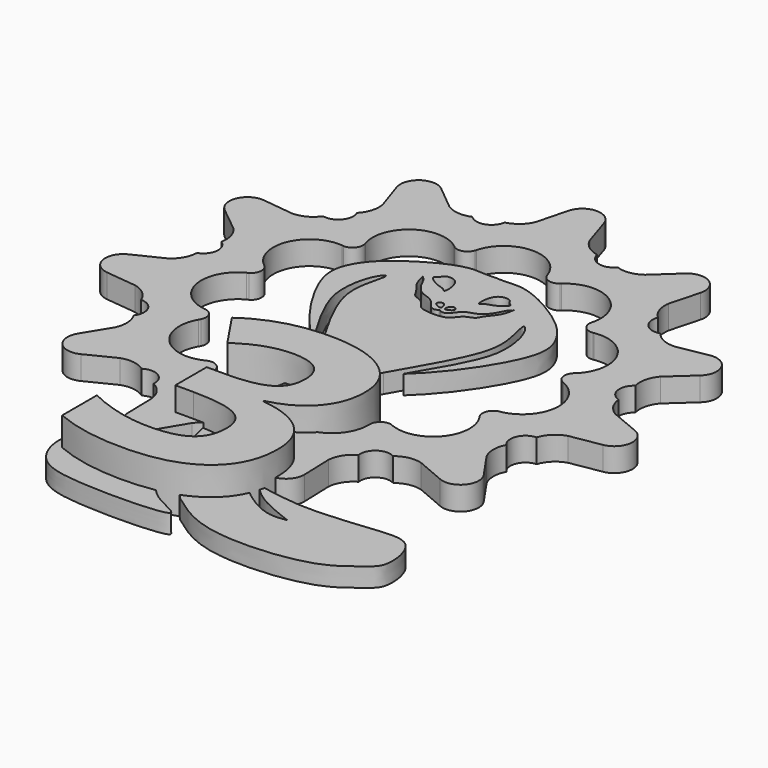
from build123d import *

# Parameters (mm, degrees)
F1_DEPTH     = 5
F3_DEPTH     = 4
F4_TEXT_SIZE = 71.6005038056
F5_DEPTH     = 10


# Not quite as in the source:
# - Text() gives the source's letters only with a copy of the font that has no kerning and outlines rounded to 1/6400 em; it was checked with that copy


with BuildPart() as f1:
    # F0 (on Top) → F1 (new body)
    with BuildSketch(Plane.XY):
        with BuildLine():
            ThreePointArc((-117.2096186083, -24.8238547917), (-113.9793205084, -29.5817996447), (-109.6649228447, -25.7793217897))
            ThreePointArc((-109.6649228447, -25.7793217897), (-109.7109933352, -25.1868355634), (-109.8480972803, -24.6085925984))
            ThreePointArc((-109.8480972803, -24.6085925984), (-113.6098018142, -21.9481109336), (-117.2096186083, -24.8238547917))
        make_face()
        with BuildLine():
            ThreePointArc((-109.8480972803, -24.6085925984), (-109.7109933352, -25.1868355634), (-109.6649228447, -25.7793217897))
            ThreePointArc((-109.6649228447, -25.7793217897), (-113.9793205084, -29.5817996447), (-117.2096186083, -24.8238547917))
            Line((-117.2096186083, -24.8238547917), (-118.8519075513, -31.2039032578))
            ThreePointArc((-118.8519075513, -31.2039032578), (-120.3942965539, -33.4215473324), (-122.7970570326, -34.6559099853))
            ThreePointArc((-122.7970570326, -34.6559099853), (-124.9522527799, -37.2281972482), (-128.2088887321, -36.4183498881))
            ThreePointArc((-128.2088887321, -36.4183498881), (-130.877743488, -36.8356308111), (-133.4302536555, -35.9515488457))
            Line((-133.4302536555, -35.9515488457), (-138.51463756, -31.7621369879))
            ThreePointArc((-138.51463756, -31.7621369879), (-143.1175497707, -31.5577284026), (-144.591163856, -35.923165977))
            Line((-144.591163856, -35.923165977), (-142.5234306131, -42.1782927254))
            ThreePointArc((-142.5234306131, -42.1782927254), (-142.6220219053, -44.8777720889), (-143.9760058128, -47.2152144208))
            ThreePointArc((-143.9760058128, -47.2152144208), (-144.3983883606, -50.5443469588), (-147.5758813994, -51.6237303294))
            ThreePointArc((-147.5758813994, -51.6237303294), (-149.595465792, -53.417661197), (-152.2207447845, -54.0539153038))
            Line((-152.2207447845, -54.0539153038), (-158.7629677579, -53.2783832483))
            ThreePointArc((-158.7629677579, -53.2783832483), (-162.7456955411, -55.594946024), (-161.6252448576, -60.0640817296))
            Line((-161.6252448576, -60.0640817296), (-156.5039801235, -64.2083282143))
            ThreePointArc((-156.5039801235, -64.2083282143), (-155.1274716666, -66.5325772424), (-155.0027986791, -69.2309778285))
            ThreePointArc((-155.0027986791, -69.2309778285), (-153.558264553, -72.2599795833), (-155.6477830895, -74.885897091))
            ThreePointArc((-155.6477830895, -74.885897091), (-156.376893344, -77.486917528), (-158.2414336307, -79.4415015236))
            Line((-158.2414336307, -79.4415015236), (-164.164386104, -82.3260752185))
            ThreePointArc((-164.164386104, -82.3260752185), (-166.2624415292, -86.428117042), (-162.9036612522, -89.5820318695))
            Line((-162.9036612522, -89.5820318695), (-156.3548303948, -90.2996291135))
            ThreePointArc((-156.3548303948, -90.2996291135), (-153.9402538979, -91.5107151622), (-152.3765068081, -93.7133508823))
            ThreePointArc((-152.3765068081, -93.7133508823), (-149.5236853864, -95.4805351987), (-149.8618220492, -98.8192765887))
            ThreePointArc((-149.8618220492, -98.8192765887), (-149.0689708113, -101.4015809842), (-149.5807940254, -104.0539282605))
            Line((-149.5807940254, -104.0539282605), (-153.003980438, -109.682775939))
            ThreePointArc((-153.003980438, -109.682775939), (-152.5512457318, -114.267927515), (-148.0205248672, -115.1052757913))
            Line((-148.0205248672, -115.1052757913), (-142.123335412, -112.1683917398))
            ThreePointArc((-142.123335412, -112.1683917398), (-139.4373018523, -111.8818035458), (-136.9309593122, -112.8893531219))
            ThreePointArc((-136.9309593122, -112.8893531219), (-133.5756012393, -112.8336514657), (-132.0550000271, -115.8251899371))
            ThreePointArc((-132.0550000271, -115.8251899371), (-129.9919119629, -117.5689148913), (-128.9885178503, -120.0769239287))
            Line((-128.9885178503, -120.0769239287), (-128.8251007032, -126.6629262244))
            ThreePointArc((-128.8251007032, -126.6629262244), (-125.965315936, -130.2754343246), (-121.7011263458, -128.5303638883))
            Line((-121.7011263458, -128.5303638883), (-118.3278942772, -122.8714384767))
            ThreePointArc((-118.3278942772, -122.8714384767), (-116.2232003313, -121.1781657666), (-113.5700083885, -120.6707393274))
            ThreePointArc((-113.5700083885, -120.6707393274), (-110.7774161447, -118.8098365809), (-107.8808571983, -120.5043798061))
            ThreePointArc((-107.8808571983, -120.5043798061), (-105.2025481911, -120.8559049667), (-103.0025072929, -122.4233006165))
            Line((-103.0025072929, -122.4233006165), (-99.3043703757, -127.8754483349))
            ThreePointArc((-99.3043703757, -127.8754483349), (-94.9454970048, -129.3683671623), (-92.3016887545, -125.594925547))
            Line((-92.3016887545, -125.594925547), (-92.5233914202, -119.0106276094))
            ThreePointArc((-92.5233914202, -119.0106276094), (-91.6682625448, -116.4482725046), (-89.7105908946, -114.586974359))
            ThreePointArc((-89.7105908946, -114.586974359), (-88.3673927857, -111.5116939958), (-85.0145131046, -111.371236474))
            ThreePointArc((-85.0145131046, -111.371236474), (-82.5713273401, -110.2189550861), (-79.8731370967, -110.3481003042))
            Line((-79.8731370967, -110.3481003042), (-73.8144127508, -112.9353750679))
            ThreePointArc((-73.8144127508, -112.9353750679), (-69.3403622731, -111.8347134433), (-69.156325802, -107.2309416998))
            Line((-69.156325802, -107.2309416998), (-72.9025741721, -101.811739309))
            ThreePointArc((-72.9025741721, -101.811739309), (-73.5685077432, -99.1938314505), (-72.9279033022, -96.5696106086))
            ThreePointArc((-72.9279033022, -96.5696106086), (-73.4605552373, -93.2563324151), (-70.7158704298, -91.325468417))
            ThreePointArc((-70.7158704298, -91.325468417), (-69.2835021255, -89.0352216797), (-66.9438188747, -87.6851137718))
            Line((-66.9438188747, -87.6851137718), (-60.4481092711, -86.5860741241))
            ThreePointArc((-60.4481092711, -86.5860741241), (-57.2793611012, -83.2412843363), (-59.6135266884, -79.2688474646))
            Line((-59.6135266884, -79.2688474646), (-65.6949133751, -76.7352990894))
            ThreePointArc((-65.6949133751, -76.7352990894), (-67.6704801891, -74.893005725), (-68.5503303411, -72.3390337622))
            ThreePointArc((-68.5503303411, -72.3390337622), (-70.7897190943, -69.8397001543), (-69.5246471938, -66.7314653564))
            ThreePointArc((-69.5246471938, -66.7314653564), (-69.5578631658, -64.0303904267), (-68.3195198083, -61.6296791142))
            Line((-68.3195198083, -61.6296791142), (-63.4491668495, -57.1932623778))
            ThreePointArc((-63.4491668495, -57.1932623778), (-62.591776142, -52.6662915513), (-66.7030627062, -50.5864101902))
            Line((-66.7030627062, -50.5864101902), (-73.1887904055, -51.7428995386))
            ThreePointArc((-73.1887904055, -51.7428995386), (-75.8467619576, -51.2611357945), (-77.967720496, -49.5882807635))
            ThreePointArc((-77.967720496, -49.5882807635), (-81.202855961, -48.6964125022), (-81.8190483573, -45.3976494912))
            ThreePointArc((-81.8190483573, -45.3976494912), (-83.3073027691, -43.1433185744), (-83.5634645712, -40.4542127364))
            Line((-83.5634645712, -40.4542127364), (-81.8647709095, -34.0889498788))
            ThreePointArc((-81.8647709095, -34.0889498788), (-83.590953156, -29.8170792651), (-88.1740562618, -30.290101051))
            Line((-88.1740562618, -30.290101051), (-93.0049522552, -34.7694509261))
            ThreePointArc((-93.0049522552, -34.7694509261), (-95.501441358, -35.8011733872), (-98.1901189329, -35.5405549404))
            ThreePointArc((-98.1901189329, -35.5405549404), (-101.3938684578, -36.5393138971), (-103.695688419, -34.097356621))
            ThreePointArc((-103.695688419, -34.097356621), (-106.1664710103, -33.0055038548), (-107.8358084098, -30.8817755946))
            Line((-107.8358084098, -30.8817755946), (-109.8480972803, -24.6085925984))
        make_face()
        with BuildLine():
            ThreePointArc((-120.2761988919, -45.2671052015), (-113.1332584373, -39.6167331027), (-105.6182130227, -44.7618662992))
            ThreePointArc((-105.6182130227, -44.7618662992), (-105.5515166298, -44.9618399206), (-105.4903344746, -45.1635689516))
            ThreePointArc((-105.4903344746, -45.1635689516), (-103.9595719314, -46.4625857559), (-102.0028203403, -46.0133621674))
            ThreePointArc((-102.0028203403, -46.0133621674), (-101.9053533079, -45.9208909988), (-101.8062833721, -45.8301392094))
            ThreePointArc((-101.8062833721, -45.8301392094), (-93.5450584899, -44.5228398864), (-88.990003067, -51.5377053996))
            ThreePointArc((-88.990003067, -51.5377053996), (-89.0431986034, -52.4400086199), (-89.2020482023, -53.3298106605))
            ThreePointArc((-89.2020482023, -53.3298106605), (-89.2540535283, -53.5340979684), (-89.3116467723, -53.7368807988))
            ThreePointArc((-89.3116467723, -53.7368807988), (-88.7261888819, -55.6572759873), (-86.8371960849, -56.3372648362))
            ThreePointArc((-86.8371960849, -56.3372648362), (-86.7052079114, -56.312167795), (-86.5728008563, -56.2893837827))
            ThreePointArc((-86.5728008563, -56.2893837827), (-80.3630657899, -58.0177108599), (-77.6577832051, -63.8682980284))
            ThreePointArc((-77.6577832051, -63.8682980284), (-78.2740870509, -66.882499127), (-80.024071995, -69.4128728916))
            ThreePointArc((-80.024071995, -69.4128728916), (-80.1782677164, -69.5566141091), (-80.3363509116, -69.6960686231))
            ThreePointArc((-80.3363509116, -69.6960686231), (-80.8820764175, -71.6281302923), (-79.6605842807, -73.2214399236))
            ThreePointArc((-79.6605842807, -73.2214399236), (-79.5359802785, -73.2716851431), (-79.4122744087, -73.3241026707))
            ThreePointArc((-79.4122744087, -73.3241026707), (-76.0493885489, -76.1557842028), (-74.79093489, -80.368113249))
            ThreePointArc((-74.79093489, -80.368113249), (-76.5425275911, -85.250019579), (-80.9982269983, -87.9047943715))
            ThreePointArc((-80.9982269983, -87.9047943715), (-81.2056570629, -87.9423526777), (-81.4140399118, -87.9742030524))
            ThreePointArc((-81.4140399118, -87.9742030524), (-82.9176848218, -89.3045152737), (-82.7515084679, -91.3052811373))
            ThreePointArc((-82.7515084679, -91.3052811373), (-82.6738495275, -91.4149161153), (-82.5981205824, -91.5258929881))
            ThreePointArc((-82.5981205824, -91.5258929881), (-81.6314443255, -93.5657632348), (-81.2996622055, -95.798576311))
            ThreePointArc((-81.2996622055, -95.798576311), (-84.6667499566, -102.1526848554), (-91.8152258815, -102.9345206881))
            ThreePointArc((-91.8152258815, -102.9345206881), (-92.0100327095, -102.8539715861), (-92.2025551299, -102.7681055526))
            ThreePointArc((-92.2025551299, -102.7681055526), (-94.1867228094, -103.0743035952), (-95.1286220566, -104.8472966661))
            ThreePointArc((-95.1286220566, -104.8472966661), (-95.1225643428, -104.9815130717), (-95.1188557274, -105.1158149169))
            ThreePointArc((-95.1188557274, -105.1158149169), (-95.1178316026, -105.1882163487), (-95.1174902175, -105.2606242187))
            ThreePointArc((-95.1174902175, -105.2606242187), (-100.449401412, -112.5721628925), (-109.0407479285, -109.7302199307))
            ThreePointArc((-109.0407479285, -109.7302199307), (-109.1610817285, -109.5571371914), (-109.2766192122, -109.3808166086))
            ThreePointArc((-109.2766192122, -109.3808166086), (-111.1113504424, -108.5656847574), (-112.8622789349, -109.5479922631))
            ThreePointArc((-112.8622789349, -109.5479922631), (-112.929745729, -109.6641773358), (-112.9992349025, -109.7791642664))
            ThreePointArc((-112.9992349025, -109.7791642664), (-121.4447298582, -113.1882577158), (-127.2058115992, -106.1343056061))
            ThreePointArc((-127.2058115992, -106.1343056061), (-127.2134672398, -105.9236417761), (-127.2153374522, -105.7128471832))
            ThreePointArc((-127.2153374522, -105.7128471832), (-128.318118031, -104.0351840417), (-130.3221683439, -103.9149302896))
            ThreePointArc((-130.3221683439, -103.9149302896), (-130.4417394155, -103.9761960899), (-130.5623640564, -104.0353605678))
            ThreePointArc((-130.5623640564, -104.0353605678), (-139.5102615936, -102.3372931793), (-140.5431375262, -93.2884551046))
            ThreePointArc((-140.5431375262, -93.2884551046), (-140.4356843958, -93.1070944616), (-140.3232935575, -92.9287516525))
            ThreePointArc((-140.3232935575, -92.9287516525), (-140.3439984431, -90.9212034142), (-141.964898762, -89.736568121))
            ThreePointArc((-141.964898762, -89.736568121), (-142.0986111407, -89.7234631901), (-142.2320737777, -89.7080209117))
            ThreePointArc((-142.2320737777, -89.7080209117), (-148.8414796513, -83.441917083), (-144.8182189649, -75.2711351962))
            ThreePointArc((-144.8182189649, -75.2711351962), (-144.629772673, -75.1766584628), (-144.4388040811, -75.0873900193))
            ThreePointArc((-144.4388040811, -75.0873900193), (-143.3708596186, -73.3873390652), (-144.093985545, -71.5144355663))
            ThreePointArc((-144.093985545, -71.5144355663), (-144.1993864954, -71.4311206271), (-144.3033136842, -71.3459744067))
            ThreePointArc((-144.3033136842, -71.3459744067), (-146.4757882291, -62.5012778294), (-138.6737477646, -57.8027176474))
            ThreePointArc((-138.6737477646, -57.8027176474), (-138.4641386775, -57.825120519), (-138.2552235106, -57.8532685411))
            ThreePointArc((-138.2552235106, -57.8532685411), (-136.4376945211, -57.0004690372), (-136.0334586827, -55.0339309601))
            ThreePointArc((-136.0334586827, -55.0339309601), (-136.0770841477, -54.9068579172), (-136.1184797403, -54.7790410781))
            ThreePointArc((-136.1184797403, -54.7790410781), (-133.1642776385, -46.1638804218), (-124.0605501168, -46.429301604))
            ThreePointArc((-124.0605501168, -46.429301604), (-123.8963276385, -46.5614713272), (-123.7357949861, -46.6980990168))
            ThreePointArc((-123.7357949861, -46.6980990168), (-121.7457340817, -46.9633087799), (-120.342478501, -45.5274980693))
            ThreePointArc((-120.342478501, -45.5274980693), (-120.3104777038, -45.3970117159), (-120.2761988919, -45.2671052015))
        make_face(mode=Mode.SUBTRACT)
    extrude(amount=F1_DEPTH)

    # F2 (on Top) → F3 (join)
    with BuildSketch(Plane.XY):
        with BuildLine():
            add(Edge.make_bspline(
                [(-112.8318831325, -49.5106913149), (-110.8358390301, -49.7867201321), (-106.8673193815, -48.3627424801), (-95.4730686789, -54.9641453728), (-91.24145791, -59.9110418173), (-88.8182301333, -66.581057202), (-97.3949212358, -80.1979328277), (-101.4951824369, -84.1600654045), (-103.252193262, -85.8743322902)],
                knots=[0, 0, 0, 0, 0.1365349459, 0.3342831137, 0.4785284841, 0.6175654811, 0.8376307999, 1, 1, 1, 1], degree=3))
            add(Edge.make_bspline(
                [(-112.8318831325, -49.5106913149), (-114.8279272348, -49.7867201321), (-118.7964468834, -48.3627424801), (-130.190697586, -54.9641453728), (-134.4223083549, -59.9110418173), (-136.8455361317, -66.581057202), (-128.2688450291, -80.1979328277), (-124.168583828, -84.1600654045), (-122.4115730029, -85.8743322902)],
                knots=[0, 0, 0, 0, 0.1365349459, 0.3342831137, 0.4785284841, 0.6175654811, 0.8376307999, 1, 1, 1, 1], degree=3))
            add(Edge.make_bspline(
                [(-122.4115730029, -85.8743322902), (-124.958112917, -81.6141024189), (-129.2089516234, -74.369457322), (-130.4225910024, -68.1737151841), (-129.3185920534, -62.1735759595), (-126.9601199795, -59.2936404783), (-127.8236442382, -63.3904845171), (-129.9288002995, -70.947818882), (-118.5329024032, -88.3060464577), (-114.9407244822, -98.0306761721), (-119.7444756613, -110.6590313317), (-116.479102874, -126.0767500088), (-113.2716186955, -132.3290730332), (-112.8318831325, -133.1038787181)],
                knots=[0, 0, 0, 0, 0.1073418359, 0.1800553274, 0.2527196236, 0.2951183014, 0.3404049451, 0.4217451234, 0.5528269749, 0.6458771787, 0.7495835625, 0.8817656203, 0.9014576568, 0.9014576568, 0.9014576568, 0.9014576568], degree=3))
            add(Edge.make_bspline(
                [(-106.4971447376, -88.3240836838), (-106.5080314354, -88.3443907053), (-108.561729288, -92.1796397896), (-110.7230417827, -98.0306761721), (-105.9192906036, -110.6590313317), (-109.184663391, -126.0767500088), (-112.3921475694, -132.3290730332), (-112.8318831325, -133.1038787181)],
                knots=[0.5523323878, 0.5523323878, 0.5523323878, 0.5523323878, 0.5528269749, 0.6458771787, 0.7495835625, 0.8817656203, 0.9014576568, 0.9014576568, 0.9014576568, 0.9014576568], degree=3))
            add(Edge.make_bspline(
                [(-106.1023806814, -87.5969630464), (-106.247526419, -87.8281931787), (-106.3789975954, -88.0715097531), (-106.4971447376, -88.3240836838)],
                knots=[0, 0, 0, 0, 0.0668727136, 0.0668727136, 0.0668727136, 0.0668727136], degree=3))
            add(Edge.make_bspline(
                [(-103.252193262, -85.8743322902), (-100.7056533479, -81.6141024189), (-96.4548146415, -74.369457322), (-95.2411752625, -68.1737151841), (-96.3451742116, -62.1735759595), (-98.7036462854, -59.2936404783), (-97.8401220267, -63.3904845171), (-95.7864452579, -70.763012523), (-103.1978484029, -82.3074697159), (-106.1023806814, -87.5969630464)],
                knots=[0, 0, 0, 0, 0.1073418359, 0.1800553274, 0.2527196236, 0.2951183014, 0.3404049451, 0.4217451234, 0.5465249907, 0.5465249907, 0.5465249907, 0.5465249907], degree=3))
        make_face()
        with BuildLine():
            add(Edge.make_bspline(
                [(-120.9213361144, -55.7986162603), (-120.9253523737, -55.5501994682), (-120.121301053, -55.2735206681), (-119.914520435, -54.0254688498), (-116.3753834879, -53.9011755123), (-116.1277862601, -59.2035980251), (-117.1620053446, -57.8149655297), (-118.6804147561, -57.7393391349), (-120.9141481965, -56.2432089485), (-120.9213361144, -55.7986162603)],
                knots=[0, 0, 0, 0, 0.0989707847, 0.2106465985, 0.3821345415, 0.5887087596, 0.6783506169, 0.8228715262, 1, 1, 1, 1], degree=3))
        make_face(mode=Mode.SUBTRACT)
        with BuildLine():
            add(Edge.make_bspline(
                [(-114.5205646753, -62.2444786131), (-114.7149933945, -62.4161081327), (-115.039833193, -62.9456021631), (-112.6423379425, -64.1385815883), (-113.5898900749, -61.7056093361), (-114.300401944, -62.0501327163), (-114.5205646753, -62.2444786131)],
                knots=[0, 0, 0, 0, 0.1930551619, 0.4930075768, 0.781392626, 1, 1, 1, 1], degree=3))
        make_face(mode=Mode.SUBTRACT)
        with BuildLine():
            add(Edge.make_bspline(
                [(-111.1432015896, -62.2444786131), (-110.9487728704, -62.4161081327), (-110.6239330719, -62.9456021631), (-113.0214283224, -64.1385815883), (-112.07387619, -61.7056093361), (-111.3633643209, -62.0501327163), (-111.1432015896, -62.2444786131)],
                knots=[0, 0, 0, 0, 0.1930551619, 0.4930075768, 0.781392626, 1, 1, 1, 1], degree=3))
        make_face(mode=Mode.SUBTRACT)
        with BuildLine():
            add(Edge.make_bspline(
                [(-122.4722117186, -56.6797964275), (-122.2710363201, -57.6203907236), (-121.8734072398, -59.4795029596), (-119.8516614569, -61.4410029015), (-119.3667720594, -63.017108625), (-117.5095003129, -63.3317861325), (-116.3789458331, -64.7651717136), (-115.5997016165, -65.8961752972), (-113.6699818537, -66.0383911582), (-112.8318831325, -66.0723300775)],
                knots=[0, 0, 0, 0, 0.1506450255, 0.2977543149, 0.406105999, 0.5214049942, 0.639197965, 0.7455654976, 0.8725879079, 0.8725879079, 0.8725879079, 0.8725879079], degree=3))
            add(Edge.make_bspline(
                [(-122.4722117186, -56.6797964275), (-122.2023545736, -56.9124290853), (-121.5648981776, -57.4619538189), (-120.8206628684, -59.4246897054), (-118.9779005615, -61.5980774521), (-116.7423323209, -61.9029688668), (-115.5246672074, -63.1222307371), (-114.8382844837, -64.2373031307), (-113.6914037557, -64.8220376107), (-113.1645601796, -64.4848196837), (-112.9202321172, -64.3284320831)],
                knots=[0, 0, 0, 0, 0.1055652862, 0.2493662598, 0.4151727066, 0.5614349786, 0.6884801018, 0.8032849912, 0.9087717889, 1, 1, 1, 1], degree=3))
            add(Edge.make_bspline(
                [(-112.9202321172, -64.3284320831), (-112.8971684193, -64.3031555502), (-112.8479666038, -64.2492330911), (-112.7797655021, -64.30095512), (-112.7435341477, -64.3284320831)],
                knots=[0, 0, 0, 0, 0.4687570504, 1, 1, 1, 1], degree=3))
            add(Edge.make_bspline(
                [(-103.1915545464, -56.6797964275), (-103.4614116913, -56.9124290853), (-104.0988680874, -57.4619538189), (-104.8431033965, -59.4246897054), (-106.6858657034, -61.5980774521), (-108.921433944, -61.9029688668), (-110.1390990575, -63.1222307371), (-110.8254817812, -64.2373031307), (-111.9723625092, -64.8220376107), (-112.4992060853, -64.4848196837), (-112.7435341477, -64.3284320831)],
                knots=[0, 0, 0, 0, 0.1055652862, 0.2493662598, 0.4151727066, 0.5614349786, 0.6884801018, 0.8032849912, 0.9087717889, 1, 1, 1, 1], degree=3))
            add(Edge.make_bspline(
                [(-103.1915545464, -56.6797964275), (-103.3927299448, -57.6203907236), (-103.7903590251, -59.4795029596), (-105.812104808, -61.4410029015), (-106.2969942055, -63.017108625), (-108.1542659521, -63.3317861325), (-109.2848204318, -64.7651717136), (-110.0640646484, -65.8961752972), (-111.9937844112, -66.0383911582), (-112.8318831325, -66.0723300775)],
                knots=[0, 0, 0, 0, 0.1506450255, 0.2977543149, 0.406105999, 0.5214049942, 0.639197965, 0.7455654976, 0.8725879079, 0.8725879079, 0.8725879079, 0.8725879079], degree=3))
        make_face(mode=Mode.SUBTRACT)
        with BuildLine():
            add(Edge.make_bspline(
                [(-104.7424301505, -55.7986162603), (-104.7384138912, -55.5501994682), (-105.5424652119, -55.2735206681), (-105.7492458299, -54.0254688498), (-109.288382777, -53.9011755123), (-109.5359800049, -59.2035980251), (-108.5017609203, -57.8149655297), (-106.9833515088, -57.7393391349), (-104.7496180684, -56.2432089485), (-104.7424301505, -55.7986162603)],
                knots=[0, 0, 0, 0, 0.0989707847, 0.2106465985, 0.3821345415, 0.5887087596, 0.6783506169, 0.8228715262, 1, 1, 1, 1], degree=3))
        make_face(mode=Mode.SUBTRACT)
        with BuildLine():
            add(Edge.make_bspline(
                [(-106.4971447376, -88.3240836838), (-106.5080314354, -88.3443907053), (-108.561729288, -92.1796397896), (-110.7230417827, -98.0306761721), (-105.9192906036, -110.6590313317), (-109.184663391, -126.0767500088), (-112.3921475694, -132.3290730332), (-112.8318831325, -133.1038787181)],
                knots=[0.5523323878, 0.5523323878, 0.5523323878, 0.5523323878, 0.5528269749, 0.6458771787, 0.7495835625, 0.8817656203, 0.9014576568, 0.9014576568, 0.9014576568, 0.9014576568], degree=3))
            add(Edge.make_bspline(
                [(-112.8318831325, -133.1038787181), (-110.6313706081, -136.9811398648), (-107.8335552111, -139.9600981471), (-104.1188687086, -143.6747908592)],
                knots=[0.9014576568, 0.9014576568, 0.9014576568, 0.9014576568, 1, 1, 1, 1], degree=3))
            add(Edge.make_bspline(
                [(-104.1188687086, -143.6747908592), (-101.1795778119, -145.8475139806), (-94.3011891386, -150.9320172276), (-71.945991858, -149.4224634712), (-65.7249745221, -143.7169190283), (-62.1329094718, -141.4398888485), (-63.6617444564, -131.6409376694), (-72.1141146769, -132.1460815159), (-85.7630138709, -133.9098409818), (-93.5349725426, -132.4330135485), (-97.2476452589, -131.7275315523)],
                knots=[0, 0, 0, 0, 0.1357922894, 0.3177746532, 0.4290345724, 0.504272094, 0.6129034486, 0.7174719205, 0.8650360435, 1, 1, 1, 1], degree=3))
            add(Edge.make_bspline(
                [(-97.2476452589, -131.7275315523), (-96.036400975, -132.934937646), (-93.3065488897, -135.6561393772), (-88.2815064014, -137.5866934813), (-85.4860916734, -138.6606544256)],
                knots=[0, 0, 0, 0, 0.4437032653, 1, 1, 1, 1], degree=3))
            add(Edge.make_bspline(
                [(-85.4860916734, -138.6606544256), (-86.8214382281, -138.8686993291), (-90.1986627031, -139.3948656172), (-99.4382452964, -133.5401724985), (-105.9898202639, -122.2936220443), (-107.8827210996, -108.9087363208), (-107.1312096745, -101.9275340585), (-106.780692935, -98.6713916063)],
                knots=[0, 0, 0, 0, 0.1323305705, 0.3346771966, 0.5653271855, 0.797261768, 1, 1, 1, 1], degree=3))
            add(Edge.make_bspline(
                [(-106.4971447376, -88.3240836838), (-107.0427153435, -89.4903997697), (-107.596191565, -92.3772290615), (-106.7896332372, -95.9788648585), (-106.7370373863, -97.8706617635), (-106.780692935, -98.6713916063)],
                knots=[0.0668727136, 0.0668727136, 0.0668727136, 0.0668727136, 0.375672285, 0.720566727, 1, 1, 1, 1], degree=3))
        make_face()
    extrude(amount=F3_DEPTH)



with BuildPart() as f3:
    # F2 (on Top) → F3, piece 2 (new body)
    with BuildSketch(Plane.XY):
        with BuildLine():
            add(Edge.make_bspline(
                [(-114.1436048406, -135.2139026393), (-113.3266834948, -136.643573923), (-111.22434222, -141.3956851453), (-107.896761029, -146.0280868241), (-96.9865458032, -149.6917955967), (-121.9202391847, -150.1579872782), (-130.2645211074, -147.7463969471), (-133.3287114446, -141.4572734317), (-132.3225696274, -133.9443087199), (-121.6918336805, -133.0431681273), (-117.786862751, -131.627024127), (-116.3815036416, -132.4970573187)],
                knots=[0.0521846679, 0.0521846679, 0.0521846679, 0.0521846679, 0.1140890373, 0.2241136411, 0.3113088143, 0.4773605409, 0.5991782782, 0.6939493717, 0.7892598474, 0.9103424309, 1, 1, 1, 1], degree=3))
            add(Edge.make_bspline(
                [(-116.3815036416, -132.4970573187), (-115.5635225254, -133.0034550902), (-114.8322600931, -134.0087062711), (-114.1436048406, -135.2139026393)],
                knots=[0, 0, 0, 0, 0.0521846679, 0.0521846679, 0.0521846679, 0.0521846679], degree=3))
        make_face()
    extrude(amount=F3_DEPTH)


with BuildPart() as f1_1:
    add(f1.part)

    add(f3.part)  # F5 merges F3
    # F4 (on Top) → F5 (join)
    with BuildSketch(Plane.XY):
        with Locations((-133.4854662418, -143.6647698283)):
            Text('3', F4_TEXT_SIZE, font='Open Sans', font_style=FontStyle.BOLD, text_align=(TextAlign.LEFT, TextAlign.BOTTOM))
    extrude(amount=F5_DEPTH)


solid = f1_1.part
